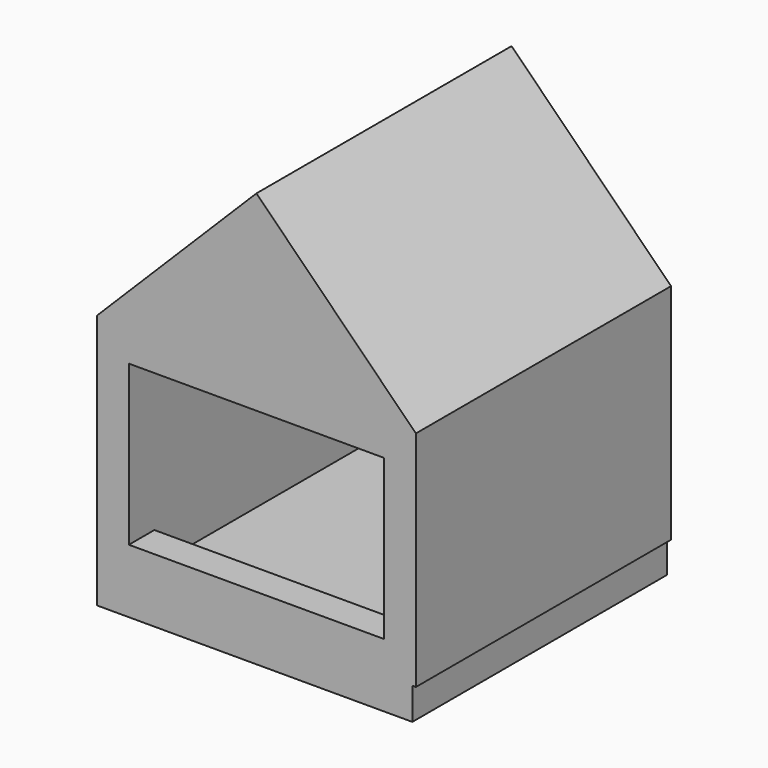
from build123d import *

# Parameters (mm, degrees)
F0_W     = 50
F0_H     = 50
F0_W_2   = 40
F0_H_2   = 40
F1_DEPTH = 35
F2_W     = 50
F2_H     = 50
F3_DEPTH = 25
F4_SIZE  = 24.99999
F5_W     = 40
F5_H     = 25
F6_DEPTH = 35
F8_W     = 49.4415648282
F8_H     = 49.9527305365
F9_DEPTH = 5


# Not quite as in the source:
# - a fillet or chamfer is up to 0.001 mm smaller than in the source, because OpenCascade refuses the exact size


with BuildPart() as f1:
    # F0 (on Top) → F1 (new body)
    with BuildSketch(Plane.XY):
        with Locations((25, 25)):
            Rectangle(F0_W, F0_H)
        with Locations((25, 25)):
            Rectangle(F0_W_2, F0_H_2, mode=Mode.SUBTRACT)
    extrude(amount=F1_DEPTH)

    # F2 (on face) → F3 (join)
    with BuildSketch(Plane.XY.offset(35)):
        with Locations((25, 25)):
            Rectangle(F2_W, F2_H)
    extrude(amount=F3_DEPTH)

    # F4 (size 25 in the source; OpenCascade refuses exactly that, so slightly less here)
    f4_edges = [f1.edges().sort_by_distance(p)[0] for p in [
        (0, 25, 60),
        (50, 25, 60),
    ]]
    chamfer(f4_edges, length=F4_SIZE)

    # F5 (on face) → F6 (cut)
    with BuildSketch(Plane.XZ):
        with Locations((25, 17.5)):
            Rectangle(F5_W, F5_H)
    extrude(amount=-F6_DEPTH, mode=Mode.SUBTRACT)

    # F8 (on face) → F9 (join)
    with BuildSketch(Plane(origin=(0, 0, 0), x_dir=(1, 0, 0), z_dir=(0, 0, -1))):
        with Locations((24.7207824141, -24.9763652682)):
            Rectangle(F8_W, F8_H)
    extrude(amount=F9_DEPTH)


solid = f1.part
